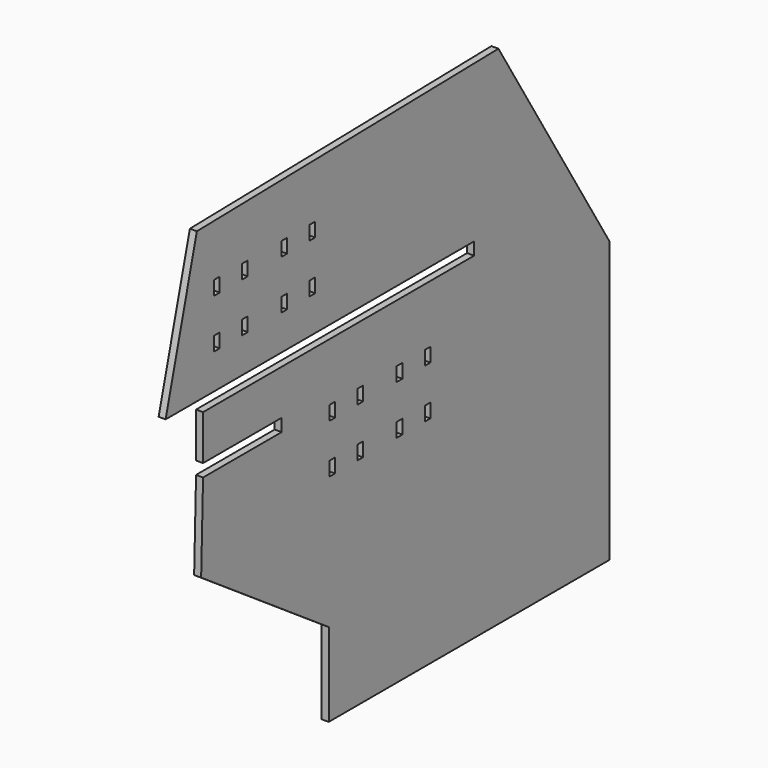
from build123d import *

# Parameters (mm, degrees)
F0_W     = 5
F0_H     = 10
F1_DEPTH = 5


# Not quite as in the source:
# - a feature names something its author has since deleted; it is built from what else it names


with BuildPart() as f1:
    # F0 (on Right) → F1 (new body)
    with BuildSketch(Plane.YZ):
        Polygon((0, 59.5256769704), (0, 0), (250, 0), (250, 200), (151.1586640426, 360.9612668205), (-117.4855289776, 355.6046891351), (-145.3168663312, 248.8862540722), (129.4880870227, 248.8862540722), (129.4880870227, 239.8862540722), (-111.9774808093, 239.8862540722), (-111.9774808093, 207.8862540722), (-41.9774808093, 207.8862540722), (-41.9774808093, 198.8862540722), (-111.9774808093, 198.8862540722), (-113.683141768, 136.7378532887), align=None)
        with Locations((3.0250263214, 158.6281073093)):
            Rectangle(F0_W, F0_H, mode=Mode.SUBTRACT)
        with Locations((28.0250263214, 158.6281073093)):
            Rectangle(F0_W, F0_H, mode=Mode.SUBTRACT)
        with Locations((63.0250263214, 158.6281073093)):
            Rectangle(F0_W, F0_H, mode=Mode.SUBTRACT)
        with Locations((88.0250263214, 158.6281073093)):
            Rectangle(F0_W, F0_H, mode=Mode.SUBTRACT)
        with Locations((3.0250263214, 193.6281073093)):
            Rectangle(F0_W, F0_H, mode=Mode.SUBTRACT)
        with Locations((28.0250263214, 193.6281073093)):
            Rectangle(F0_W, F0_H, mode=Mode.SUBTRACT)
        with Locations((-99.690104425, 278.8862540722)):
            Rectangle(F0_W, F0_H, mode=Mode.SUBTRACT)
        with Locations((-99.690104425, 313.8862540722)):
            Rectangle(F0_W, F0_H, mode=Mode.SUBTRACT)
        with Locations((-74.690104425, 278.8862540722)):
            Rectangle(F0_W, F0_H, mode=Mode.SUBTRACT)
        with Locations((-74.690104425, 313.8862540722)):
            Rectangle(F0_W, F0_H, mode=Mode.SUBTRACT)
        with Locations((-39.690104425, 278.8862540722)):
            Rectangle(F0_W, F0_H, mode=Mode.SUBTRACT)
        with Locations((-14.690104425, 278.8862540722)):
            Rectangle(F0_W, F0_H, mode=Mode.SUBTRACT)
        with Locations((-39.690104425, 313.8862540722)):
            Rectangle(F0_W, F0_H, mode=Mode.SUBTRACT)
        with Locations((-14.690104425, 313.8862540722)):
            Rectangle(F0_W, F0_H, mode=Mode.SUBTRACT)
        with Locations((63.0250263214, 193.6281073093)):
            Rectangle(F0_W, F0_H, mode=Mode.SUBTRACT)
        with Locations((88.0250263214, 193.6281073093)):
            Rectangle(F0_W, F0_H, mode=Mode.SUBTRACT)
    extrude(amount=F1_DEPTH)


solid = f1.part
